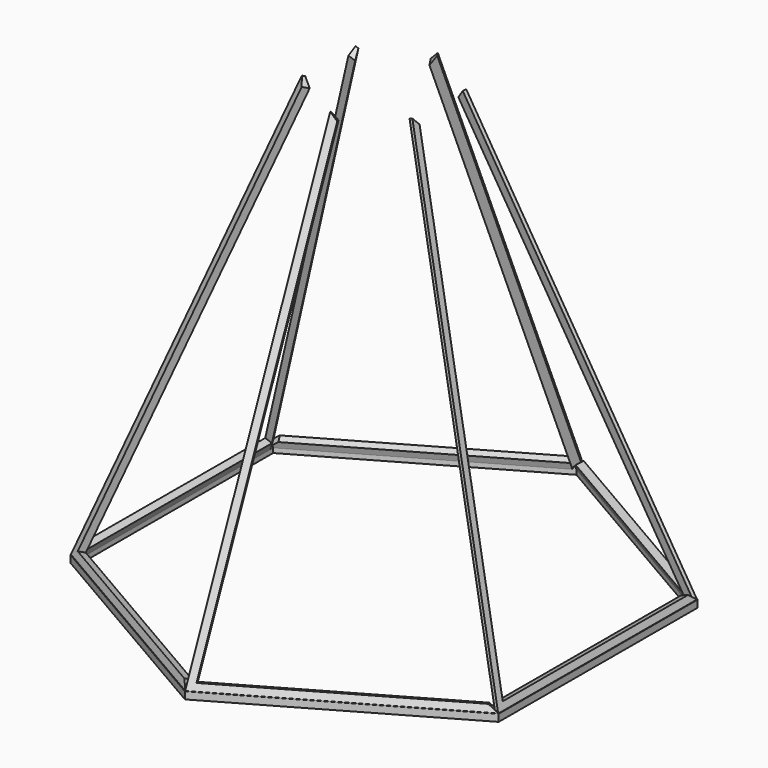
from build123d import *

# Parameters (mm, degrees)
F1_DEPTH    = 25.4
F7_DEPTH    = 25.4
F9_T1_DEPTH = 1797.8062302012
F10_COUNT   = 6


# Not quite as in the source:
# - a fillet or chamfer that OpenCascade refuses, or shapes differently, is made with other operations: its cross-section is extruded or revolved along the edge and cut away or added
# - a feature names something its author has since deleted; it is built from what else it names


with BuildPart() as f1:
    # F0 (on Top) → F1 (new body)
    with BuildSketch(Plane.XY):
        Polygon((2.5230003414, 850.548674564), (2.6100003532, 879.8779392042), (-760.6916474037, 442.1992962118), (-735.3352591569, 427.4593196714), align=None)
        Polygon((763.3016477569, 437.6786429923), (2.6100003532, 879.8779392042), (2.5230003414, 850.548674564), (737.8582594983, 423.0893548926), align=None)
        Polygon((760.6916474037, -442.1992962118), (763.3016477569, 437.6786429923), (737.8582594983, 423.0893548926), (735.3352591569, -427.4593196714), align=None)
        Polygon((-735.3352591569, 427.4593196714), (-760.6916474037, 442.1992962118), (-763.3016477569, -437.6786429923), (-737.8582594983, -423.0893548926), align=None)
        Polygon((-2.6100003532, -879.8779392042), (760.6916474037, -442.1992962118), (735.3352591569, -427.4593196714), (-2.5230003414, -850.548674564), align=None)
        Polygon((-737.8582594983, -423.0893548926), (-763.3016477569, -437.6786429923), (-2.6100003532, -879.8779392042), (-2.5230003414, -850.548674564), align=None)
    extrude(amount=F1_DEPTH)


with BuildPart() as f7:
    # F5 (on face) → F7 (new body)
    with BuildSketch(Plane(origin=(-679.5031182455, 2.0156243265, 247.319997217), x_dir=(0.0026193144, 0.9999961151, -0.0009533567), z_dir=(0.9396884866, -0.0027874176, -0.3420201433))):
        Polygon((409.3424550737, -210.9359705041), (440.1808724611, -236.3046967216), (118.6393087725, 1408.9697432491), (97.7227957299, 1383.5697432491), align=None)
        Polygon((-439.7004849555, -237.1973728844), (440.1808724611, -236.3046967216), (409.3424550737, -210.9359705041), (-408.9376758483, -211.7661496655), align=None)
    extrude(amount=F7_DEPTH)

    # F8: cut F1
    add(f1.part, mode=Mode.SUBTRACT)

    # F9: chamfer of 25.4 x 14.6646968374 on 1 edges, made by hand

    # F9_s2 → F9_t1 (cut)
    with BuildSketch(Plane(origin=(-124.6963006783, 71.3588384461, -343.1803279571), x_dir=(0.4966835337, 0.8679317182, 0), z_dir=(0.3351687947, -0.1918040531, 0.9224278206))):
        Polygon((11.7114269241, 810.4766385443), (-3.9757372853, 785.6950685295), (18.520370461, 797.4885046813), align=None)
    extrude(amount=F9_T1_DEPTH, mode=Mode.SUBTRACT)


with BuildPart() as f10_1:
    # F10: instance of F7
    add(f7.part.rotate(Axis((0, 0, 6.9533996284), (0, 0, 1)), 1 * 360 / F10_COUNT))


with BuildPart() as f10_2:
    # F10: instance of F7
    add(f7.part.rotate(Axis((0, 0, 6.9533996284), (0, 0, 1)), 2 * 360 / F10_COUNT))


with BuildPart() as f10_3:
    # F10: instance of F7
    add(f7.part.rotate(Axis((0, 0, 6.9533996284), (0, 0, 1)), 3 * 360 / F10_COUNT))


with BuildPart() as f10_4:
    # F10: instance of F7
    add(f7.part.rotate(Axis((0, 0, 6.9533996284), (0, 0, 1)), 4 * 360 / F10_COUNT))


with BuildPart() as f10_5:
    # F10: instance of F7
    add(f7.part.rotate(Axis((0, 0, 6.9533996284), (0, 0, 1)), 5 * 360 / F10_COUNT))


solid = Compound([f1.part, f7.part, f10_1.part, f10_2.part, f10_3.part, f10_4.part, f10_5.part])
